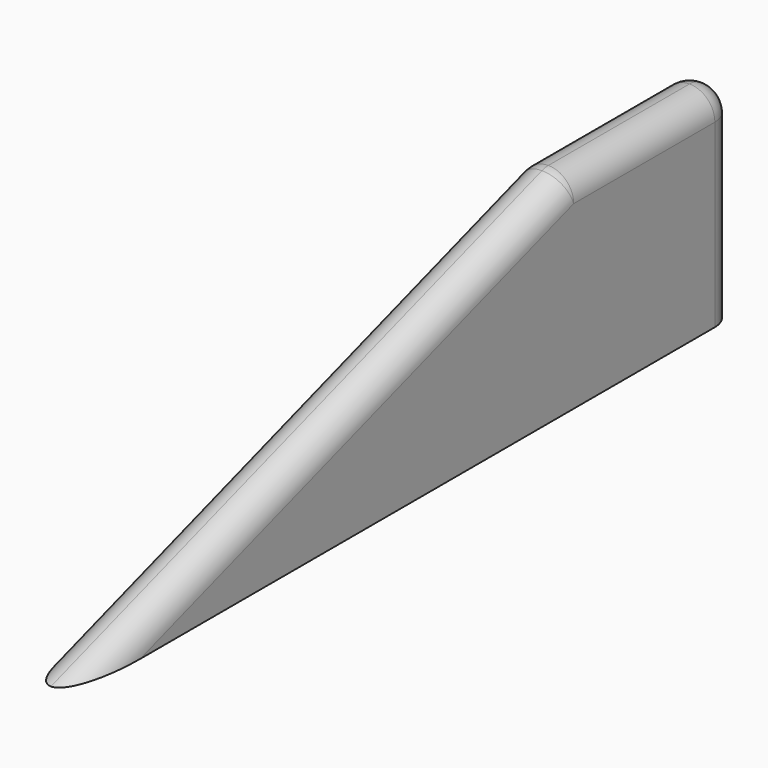
from build123d import *

# Parameters (mm, degrees)
F1_DEPTH = 0.8
F2_R     = 0.79999


# Not quite as in the source:
# - a fillet or chamfer is up to 0.001 mm smaller than in the source, because OpenCascade refuses the exact size


with BuildPart() as f1:
    # F0 (on Right) → F1 (new body, symmetric)
    with BuildSketch(Plane.YZ):
        Polygon((19.5, 6.5), (0, 0), (26, 0), (26, 6.5), align=None)
    extrude(amount=F1_DEPTH, both=True)

    # F2 (radius 0.8 in the source; OpenCascade refuses exactly that, so slightly less here)
    f2_edges = [f1.edges().sort_by_distance(p)[0] for p in [
        (0.8, 22.75, 6.5),
        (0.8, 9.75, 3.25),
        (-0.8, 22.75, 6.5),
        (-0.8, 9.75, 3.25),
        (0, 19.5, 6.5),
        (0, 26, 6.5),
        (0.8, 26, 3.25),
        (-0.8, 26, 3.25),
    ]]
    fillet(f2_edges, radius=F2_R)


solid = f1.part
